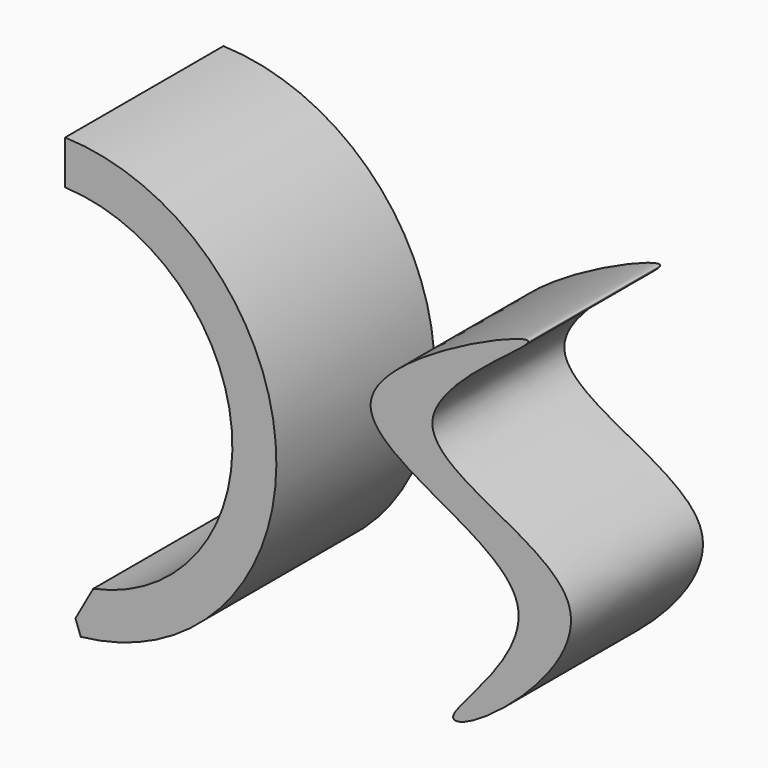
from build123d import *

# Parameters (mm, degrees)
F1_DEPTH    = 30
F3_DEPTH    = 25
F4_T1_DEPTH = 53.5744264442


# Not quite as in the source:
# - a fillet or chamfer that OpenCascade refuses, or shapes differently, is made with other operations: its cross-section is extruded or revolved along the edge and cut away or added


with BuildPart() as f1:
    # F0 (on Front) → F1 (new body)
    with BuildSketch(Plane.XZ):
        with BuildLine():
            ThreePointArc((-16.6409582285, -32.8538838982), (12.9980630113, 1.1851974836), (-19.0061628819, 33.010661602))
            Line((-19.0061628819, 33.010661602), (-19.0061628819, 26.3418406248))
            ThreePointArc((-19.0061628819, 26.3418406248), (6.3543491175, 0), (-19.0061628819, -26.3418406248))
            Line((-19.0061628819, -26.3418406248), (-16.6409582285, -32.8538838982))
        make_face()
    extrude(amount=F1_DEPTH)

    # F4: chamfer of 5 on 1 edges, made by hand

    # F4_s2 → F4_t1 (cut)
    with BuildSketch(Plane.XZ.offset(-11.7872132221)):
        with BuildLine():
            Line((-14.6446503408, -25.6553982115), (-17.5397526272, -30.822887852))
            Line((-17.5397526272, -30.822887852), (-17.6337449938, -30.8570263203))
            ThreePointArc((-17.6337449938, -30.8570263203), (-18.2957757245, -28.5906518321), (-19.1001552485, -26.3759790931))
            Line((-19.1001552485, -26.3759790931), (-19.0099575843, -26.2419126496))
            ThreePointArc((-19.0099575843, -26.2419126496), (-16.8171091828, -26.0664335828), (-14.664619643, -25.5574123606))
            Line((-14.664619643, -25.5574123606), (-14.6446503408, -25.6553982115))
        make_face()
    extrude(amount=F4_T1_DEPTH, mode=Mode.SUBTRACT)


with BuildPart() as f3:
    # F2 (on Front) → F3 (new body)
    with BuildSketch(Plane.XZ):
        with BuildLine():
            add(Edge.make_bspline(
                [(47.1818894148, 25.3415182233), (47.9254327879, 24.5473947838), (16.0534465301, 6.0583152168), (68.6264628565, -3.8046073263), (39.7238119127, -29.0846751765), (32.8029461038, -29.1373721142), (60.5747190986, -5.8473305783), (1.8881016249, 6.6933279117), (46.3185796912, 26.2635552043), (47.1818894148, 25.3415182233)],
                knots=[0, 0, 0, 0, 0.1452057039, 0.3095496455, 0.468709899, 0.5168545878, 0.6598315714, 0.8314052675, 1, 1, 1, 1], degree=3))
        make_face()
    extrude(amount=F3_DEPTH)


solid = Compound([f1.part, f3.part])
